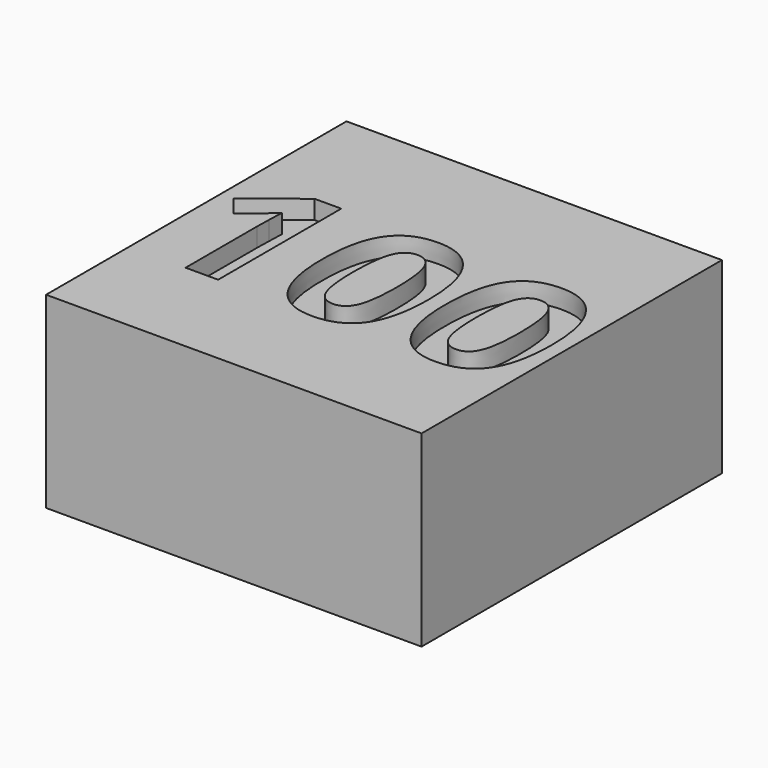
from build123d import *

# Parameters (mm, degrees)
F0_W         = 20
F0_H         = 20
F1_DEPTH     = 10
F2_TEXT_SIZE = 11.4839404271
F3_DEPTH     = 1


# Not quite as in the source:
# - Text() gives the source's letters only with a copy of the font that has no kerning and outlines rounded to 1/6400 em; it was checked with that copy


with BuildPart() as f1:
    # F0 (on Top) → F1 (new body)
    with BuildSketch(Plane.XY):
        with Locations((10, 10)):
            Rectangle(F0_W, F0_H)
    extrude(amount=F1_DEPTH)

    # F2 (on face) → F3 (cut)
    with BuildSketch(Plane.XY.offset(10)):
        with Locations((0, 5.5253425795)):
            Text('100', F2_TEXT_SIZE, font='Open Sans', font_style=FontStyle.BOLD, text_align=(TextAlign.LEFT, TextAlign.BOTTOM))
    extrude(amount=-F3_DEPTH, mode=Mode.SUBTRACT)


solid = f1.part
